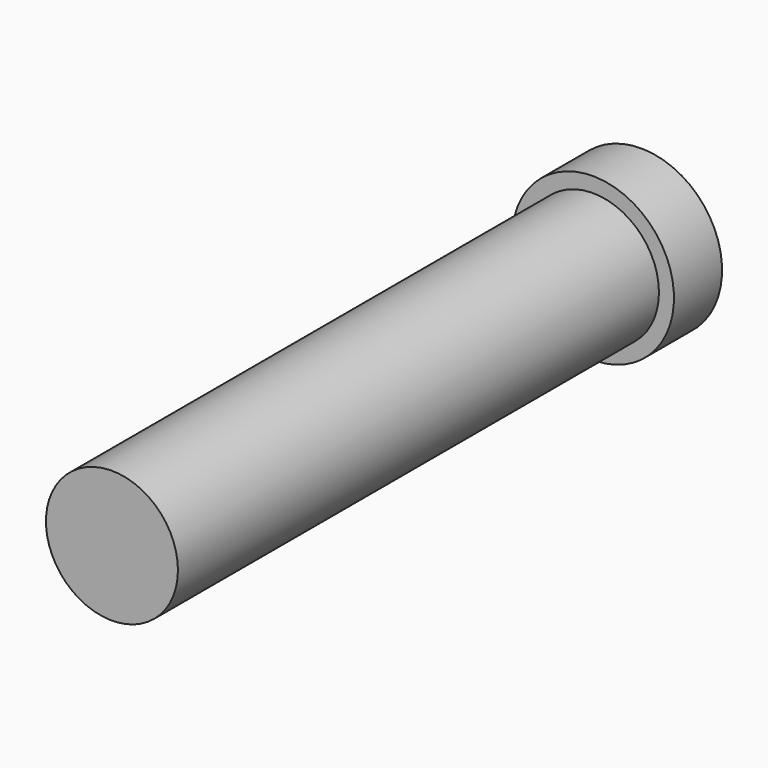
from build123d import *

# Parameters (mm, degrees)
F0_R     = 27.8765
F1_DEPTH = 254
F2_R     = 34.2265010133
F2_R_2   = 27.8765
F3_DEPTH = 25.4


with BuildPart() as f1:
    # F0 (on Front) → F1 (new body)
    with BuildSketch(Plane.XZ):
        with Locations((-2.4765, 51.8050380051)):
            Circle(F0_R)
    extrude(amount=F1_DEPTH)

    # F2 (on face) → F3 (join)
    with BuildSketch(Plane(origin=(0, 0, 0), x_dir=(-1, 0, 0), z_dir=(0, 1, 0))):
        with Locations((2.4765, 51.8050380051)):
            Circle(F2_R)
        with Locations((2.4765, 51.8050380051)):
            Circle(F2_R_2, mode=Mode.SUBTRACT)
        with Locations((2.4765, 51.8050380051)):
            Circle(F2_R_2)
    extrude(amount=F3_DEPTH)


solid = f1.part
